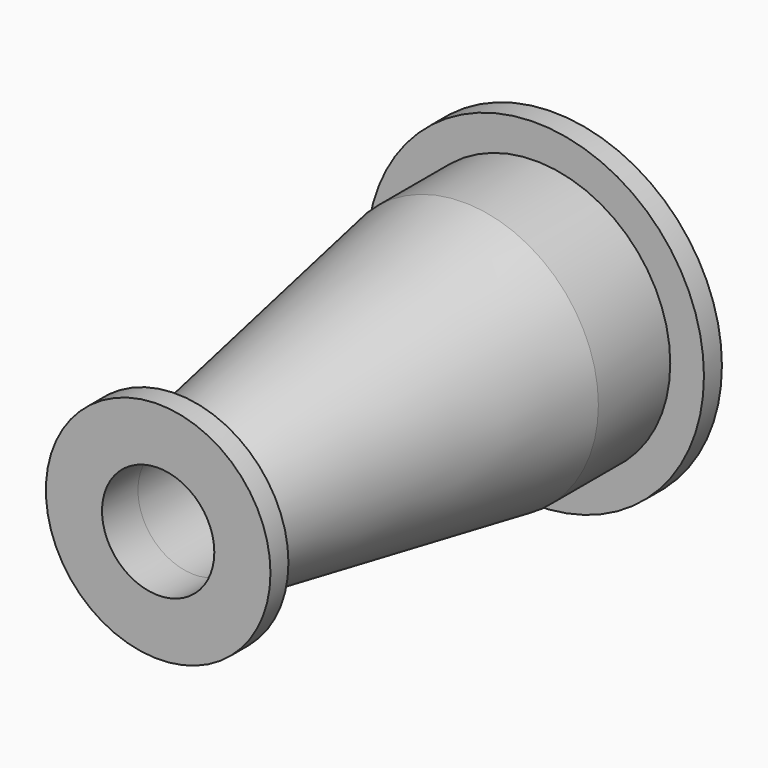
from build123d import *

# Parameters (mm, degrees)
F0_R      = 15.24
F0_R_2    = 12.7
F1_DEPTH  = 12.7
F0_R_3    = 19.05
F2_DEPTH  = 2.54
F5_R      = 15.24
F4_R      = 8.89
F7_R      = 8.89
F7_R_2    = 6.35
F8_DEPTH  = 2.54
F9_R      = 12.7
F9_R_2    = 6.35
F10_DEPTH = 2.54
F11_DEPTH = 41.402


# Not quite as in the source:
# - a fillet or chamfer that OpenCascade refuses, or shapes differently, is made with other operations: its cross-section is extruded or revolved along the edge and cut away or added


with BuildPart() as f1:
    # F0 (on Front) → F1 (new body)
    with BuildSketch(Plane.XZ):
        Circle(F0_R)
        Circle(F0_R_2, mode=Mode.SUBTRACT)
    extrude(amount=F1_DEPTH)

    # F0 (on Front) → F2 (join)
    with BuildSketch(Plane.XZ):
        Circle(F0_R_3)
        Circle(F0_R, mode=Mode.SUBTRACT)
    extrude(amount=F2_DEPTH)

    # F5 (on face) → F6 section 0
    with BuildSketch(Plane.XZ.offset(12.7)):
        Circle(F5_R)
    # F4 (on offset) → F6 section 1
    with BuildSketch(Plane.XZ.offset(50.8)):
        Circle(F4_R)
    loft()

    # F7 (on face) → F8 (join)
    with BuildSketch(Plane.XZ.offset(50.8)):
        Circle(F7_R)
        Circle(F7_R_2, mode=Mode.SUBTRACT)
    extrude(amount=F8_DEPTH)

    # F9 (on face) → F10 (join)
    with BuildSketch(Plane.XZ.offset(53.34)):
        Circle(F9_R)
        Circle(F9_R_2, mode=Mode.SUBTRACT)
    extrude(amount=F10_DEPTH)

    # F11 (cut): a face of the model
    f11_faces = [f1.faces().sort_by_distance(p)[0] for p in [
        (0, -50.8, 0),
    ]]
    extrude(f11_faces, amount=-F11_DEPTH, mode=Mode.SUBTRACT)

    # F12: fillet of radius 25.4 on 1 edges, made by hand

    # F12_s1 → F12_t2 (revolve, cut)
    with BuildSketch(Plane.XY):
        with BuildLine():
            ThreePointArc((12.7, -12.7), (7.990475594, -20.5202647042), (6.35, -29.5005208253))
            Line((6.35, -29.5005208253), (5.842, -29.5005208253))
            Line((5.842, -29.5005208253), (5.842, -12.7))
            Line((5.842, -12.7), (6.35, -12.192))
            ThreePointArc((6.35, -12.192), (9.525, -12.192), (12.319, -12.3639895835))
            Line((12.319, -12.3639895835), (12.7, -12.7))
        make_face()
    revolve(axis=Axis((0, -12.7, 0), (0, -1, 0)), mode=Mode.SUBTRACT)


solid = f1.part
